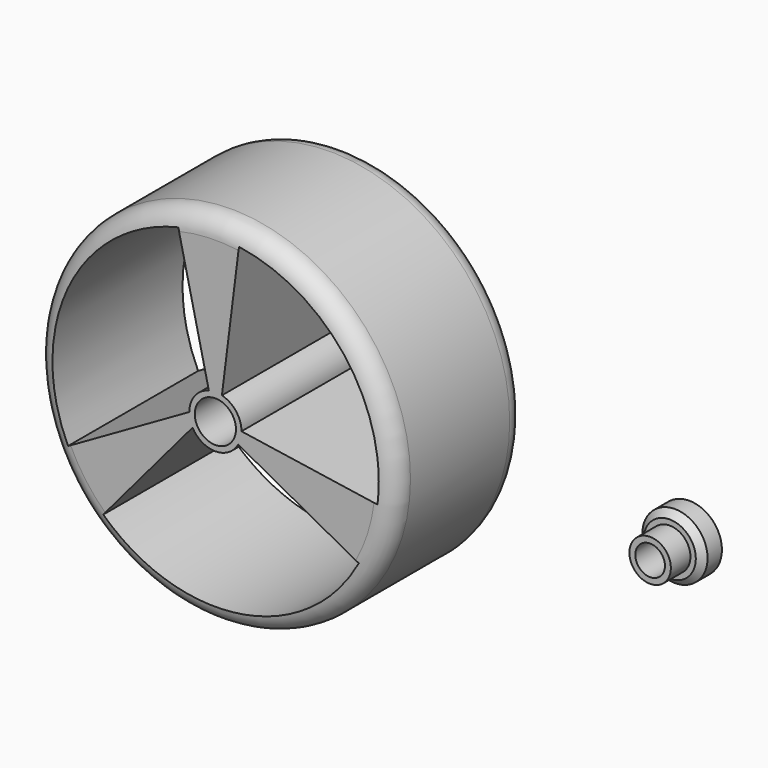
from build123d import *

# Parameters (mm, degrees)
F0_R     = 13.97
F0_R_2   = 1.6002
F1_DEPTH = 12.7
F3_R     = 1.6129
F3_R_2   = 1.1530042691
F4_DEPTH = 3.81
F3_R_3   = 2.54
F5_DEPTH = 1.905
F6_SIZE  = 0.508


# Not quite as in the source:
# - a fillet or chamfer that OpenCascade refuses, or shapes differently, is made with other operations: its cross-section is extruded or revolved along the edge and cut away or added


with BuildPart() as f1:
    # F0 (on Front) → F1 (new body)
    with BuildSketch(Plane.XZ):
        Circle(F0_R)
        with BuildLine():
            ThreePointArc((12.7, 0), (12.6753175523, -0.7914069427), (12.6013661498, -1.5797376868))
            ThreePointArc((12.6013661498, -1.5797376868), (12.0880096107, -3.894871455), (11.1532043579, -6.0742104466))
            ThreePointArc((11.1532043579, -6.0742104466), (1.9811025721, -12.5445299872), (-8.7385473465, -9.215627503))
            ThreePointArc((-8.7385473465, -9.215627503), (-10.2909600249, -7.4421866253), (-11.4889360845, -5.4124253016))
            ThreePointArc((-11.4889360845, -5.4124253016), (-11.4322745724, 5.5311027925), (-2.8867102521, 12.3675746984))
            ThreePointArc((-2.8867102521, 12.3675746984), (-0.5369932074, 12.6886420982), (1.8314490307, 12.5672508707))
            ThreePointArc((1.8314490307, 12.5672508707), (9.6059721707, 8.3075446827), (12.7, 0))
        make_face(mode=Mode.SUBTRACT)
        with BuildLine():
            ThreePointArc((1.778, -0.9837377699), (1.9674755399, -0.508), (2.032, 0))
            ThreePointArc((2.032, 0), (1.6064370514, 1.2443407893), (0.508, 1.9674755399))
            ThreePointArc((0.508, 1.9674755399), (0, 2.032), (-0.508, 1.9674755399))
            ThreePointArc((-0.508, 1.9674755399), (-1.6064370514, 1.2443407893), (-2.032, 0))
            ThreePointArc((-2.032, 0), (-1.9674755399, -0.508), (-1.778, -0.9837377699))
            ThreePointArc((-1.778, -0.9837377699), (0, -2.032), (1.778, -0.9837377699))
        make_face()
        Circle(F0_R_2, mode=Mode.SUBTRACT)
        with BuildLine():
            Line((-8.7385473465, -9.215627503), (-1.778, -0.9837377699))
            ThreePointArc((-1.778, -0.9837377699), (-1.9674755399, -0.508), (-2.032, 0))
            Line((-2.032, 0), (-11.4889360845, -5.4124253016))
            ThreePointArc((-11.4889360845, -5.4124253016), (-10.2909600249, -7.4421866253), (-8.7385473465, -9.215627503))
        make_face()
        with BuildLine():
            Line((12.6013661498, -1.5797376868), (2.032, 0))
            ThreePointArc((2.032, 0), (1.9674755399, -0.508), (1.778, -0.9837377699))
            Line((1.778, -0.9837377699), (11.1532043579, -6.0742104466))
            ThreePointArc((11.1532043579, -6.0742104466), (12.0880096107, -3.894871455), (12.6013661498, -1.5797376868))
        make_face()
        with BuildLine():
            ThreePointArc((-0.508, 1.9674755399), (0, 2.032), (0.508, 1.9674755399))
            Line((0.508, 1.9674755399), (1.8314490307, 12.5672508707))
            ThreePointArc((1.8314490307, 12.5672508707), (-0.5369932074, 12.6886420982), (-2.8867102521, 12.3675746984))
            Line((-2.8867102521, 12.3675746984), (-0.508, 1.9674755399))
        make_face()
    extrude(amount=F1_DEPTH)

    # F2: fillet of radius 1.524 on 2 edges, made by hand

    # F2_s1 → F2_t2 (revolve, cut)
    with BuildSketch(Plane.XY):
        with BuildLine():
            ThreePointArc((13.97, -11.176), (13.5236307345, -12.2536307345), (12.446, -12.7))
            Line((12.446, -12.7), (13.97, -12.7))
            Line((13.97, -12.7), (13.97, -11.176))
        make_face()
    revolve(axis=Axis((0, -12.7, 0), (0, -1, 0)), mode=Mode.SUBTRACT)

    # F2_s3 → F2_t4 (revolve, cut)
    with BuildSketch(Plane.XY):
        with BuildLine():
            ThreePointArc((13.97, -1.524), (13.5236307345, -0.4463692655), (12.446, 0))
            Line((12.446, 0), (13.97, 0))
            Line((13.97, 0), (13.97, -1.524))
        make_face()
    revolve(axis=Axis((0, 0, 0), (0, -1, 0)), mode=Mode.SUBTRACT)


with BuildPart() as f4:
    # F3 (on Front) → F4 (new body)
    with BuildSketch(Plane.XZ):
        with Locations((26.7274966631, -4.4241022947)):
            Circle(F3_R)
        with Locations((26.7274966631, -4.4241022947)):
            Circle(F3_R_2, mode=Mode.SUBTRACT)
    extrude(amount=F4_DEPTH)

    # F3 (on Front) → F5 (join)
    with BuildSketch(Plane.XZ):
        with Locations((26.7274966631, -4.4241022947)):
            Circle(F3_R_3)
        with Locations((26.7274966631, -4.4241022947)):
            Circle(F3_R, mode=Mode.SUBTRACT)
    extrude(amount=F5_DEPTH)

    # F6
    f6_edges = [f4.edges().sort_by_distance(p)[0] for p in [
        (24.187497, -1.905, -4.424102),
    ]]
    chamfer(f6_edges, length=F6_SIZE)


solid = Compound([f1.part, f4.part])
